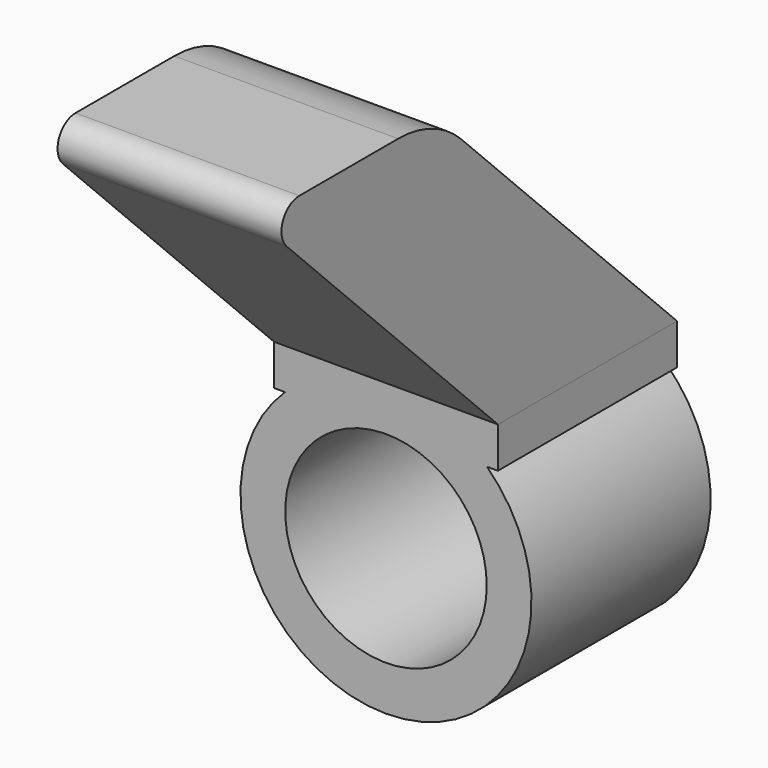
from build123d import *

# Parameters (mm, degrees)
F0_R          = 32.5
F0_R_2        = 22.5
F1_DEPTH      = 50
F3_DEPTH      = 25
F3_DEPTH_BACK = 25
F4_DEPTH      = 9.1


with BuildPart() as f1:
    # F0 (on Front) → F1 (new body)
    with BuildSketch(Plane.XZ):
        Circle(F0_R)
        Circle(F0_R_2, mode=Mode.SUBTRACT)
    extrude(amount=F1_DEPTH)



with BuildPart() as f3:
    # F2 (on Right) → F3 (new body, two sides)
    with BuildSketch(Plane.YZ) as f3_sk:
        with BuildLine():
            Line((-50, 32.5), (0, 32.5))
            Line((0, 32.5), (-60.1776695297, 92.6776695297))
            ThreePointArc((-60.1776695297, 92.6776695297), (-68.2882532502, 98.0969883128), (-77.8553390593, 100))
            Line((-77.8553390593, 100), (-105.4289321881, 100))
            ThreePointArc((-105.4289321881, 100), (-110.0483298507, 96.9134171618), (-108.9644660941, 91.4644660941))
            Line((-108.9644660941, 91.4644660941), (-50, 32.5))
        make_face()
    extrude(amount=F3_DEPTH)
    extrude(f3_sk.sketch, amount=-F3_DEPTH_BACK)


with BuildPart() as f1_1:
    add(f1.part)
    # F4 (add): a face of the model
    f4_faces = [f3.part.faces().sort_by_distance(p)[0] for p in [
        (0, -25, 32.5),
    ]]
    extrude(f4_faces, amount=F4_DEPTH)


solid = Compound([f3.part, f1_1.part])
